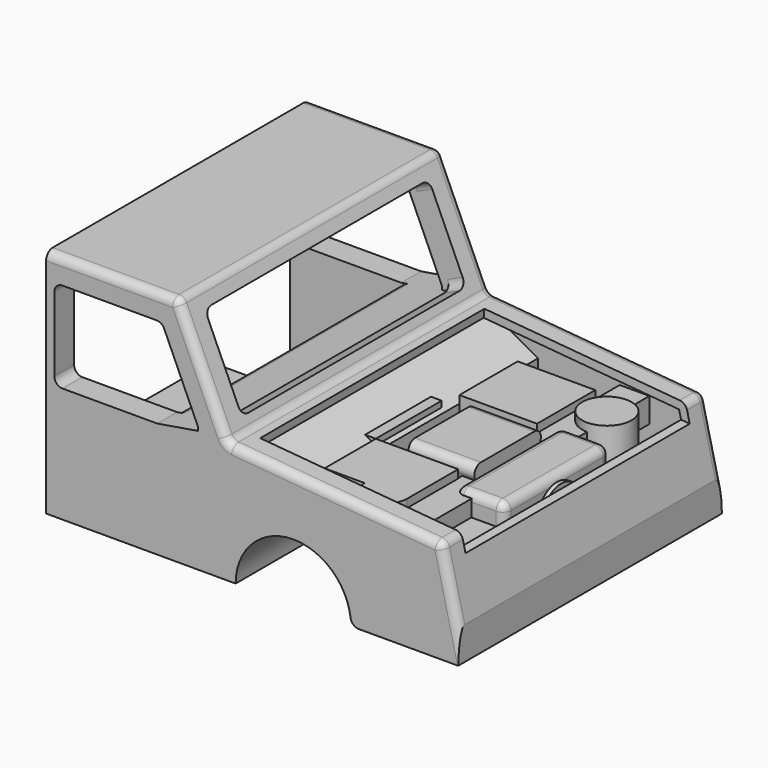
from build123d import *

# Parameters (mm, degrees)
F1_DEPTH       = 1000
F3_DEPTH       = 850
F4_W           = 1500
F4_H           = 1700
F5_DEPTH       = 100
F7_DEPTH       = 950
F9_DEPTH       = 400
F10_R          = 50
F11_R          = 150
F12_DEPTH      = 25
F13_R          = 50
F15_DEPTH      = 270
F17_DEPTH      = 1000
F18_W          = 600
F18_H          = 250
F19_DEPTH      = 250
F20_R          = 350
F21_DEPTH      = 1310
F22_R          = 50
F24_DEPTH      = 1380
F26_DEPTH      = 400
F28_DEPTH      = 150
F29_R          = 105
F30_DEPTH      = 1225
F30_DEPTH_BACK = 25
F31_W          = 180
F31_H          = 150
F32_DEPTH      = 1950
F33_R          = 150
F33_W          = 470.87931633
F33_H          = 441.7398571968
F34_DEPTH      = 180
F34_DEPTH_BACK = 50
F35_W          = 455.6799697876
F35_H          = 409.935683012
F36_DEPTH      = 100
F36_DEPTH_BACK = 50


with BuildPart() as f1:
    # F0 (on Front) → F1 (new body, symmetric)
    with BuildSketch(Plane.XZ):
        with BuildLine():
            Line((767.6470588235, 1700), (0, 1700))
            Line((0, 1700), (0, 300))
            Line((0, 300), (1103.1373033403, 300))
            ThreePointArc((1103.1373033403, 300), (1136.2091947286, 312.5), (1152.7451404228, 343.75))
            ThreePointArc((1152.7451404228, 343.75), (1500, 650), (1847.2548595772, 343.75))
            ThreePointArc((1847.2548595772, 343.75), (1863.7908052714, 312.5), (1896.8626966597, 300))
            Line((1896.8626966597, 300), (2500, 300))
            Line((2500, 300), (2500, 500))
            Line((2500, 500), (2408.3761577886, 883.3611142393))
            ThreePointArc((2408.3761577886, 883.3611142393), (2392.4030745749, 909.6000062773), (2364.1035813021, 921.5481242564))
            Line((2364.1035813021, 921.5481242564), (1129.229325017, 1029.5856225614))
            ThreePointArc((1129.229325017, 1029.5856225614), (1104.6193241933, 1038.6416182431), (1087.9773560568, 1058.9075525879))
            Line((1087.9773560568, 1058.9075525879), (813.2568149211, 1670.487804878))
            ThreePointArc((813.2568149211, 1670.487804878), (794.8096227314, 1691.9785078576), (767.6470588235, 1700))
        make_face()
        with BuildLine():
            ThreePointArc((50, 1500), (64.6446609407, 1535.3553390593), (100, 1550))
            Line((100, 1550), (670.5882352941, 1550))
            ThreePointArc((670.5882352941, 1550), (697.750799202, 1541.9785078576), (716.1979913917, 1520.487804878))
            Line((716.1979913917, 1520.487804878), (918.3370288248, 1070.487804878))
            ThreePointArc((918.3370288248, 1070.487804878), (914.7057805849, 1022.8374360921), (872.7272727273, 1000))
            Line((872.7272727273, 1000), (100, 1000))
            ThreePointArc((100, 1000), (64.6446609407, 1014.6446609407), (50, 1050))
            Line((50, 1050), (50, 1500))
        make_face(mode=Mode.SUBTRACT)
    extrude(amount=F1_DEPTH, both=True)

    # F2 (on Front) → F3 (cut, symmetric)
    with BuildSketch(Plane.XZ):
        Polygon((735.2941176471, 1600), (0, 1600), (0, 300), (2444.9838573448, 300), (2319.4915883295, 825.0691841445), (1032.8257756913, 937.6378564967), align=None)
    extrude(amount=F3_DEPTH, both=True, mode=Mode.SUBTRACT)

    # F4 (on face) → F5 (cut)
    with BuildSketch(Plane(origin=(97.9705989607, 0, 1119.8090702535), x_dir=(0.9961946981, 0, -0.0871557427), z_dir=(0.0871557427, 0, 0.9961946981))):
        with Locations((1835.197966855, 0)):
            Rectangle(F4_W, F4_H)
    extrude(amount=-F5_DEPTH, mode=Mode.SUBTRACT)

    # F6 (on Front) → F7 (cut, symmetric)
    with BuildSketch(Plane.XZ):
        Polygon((2359.7457941648, 871.7383893518), (1110.5418587764, 981.0295721303), (1110.5418587764, 281.0295721303), (2410.5418587764, 281.0295721303), (2410.5418587764, 450), (2460.5418587764, 450), align=None)
    extrude(amount=F7_DEPTH, both=True, mode=Mode.SUBTRACT)

    # F13
    f13_edges = [f1.edges().sort_by_distance(p)[0] for p in [
        (950.617085, -1000, 1364.697679),
        (1746.666453, 1000, 975.566873),
    ]]
    fillet(f13_edges, radius=F13_R)

    # F14 (on face) → F15 (cut)
    with BuildSketch(Plane(origin=(1301.1017251636, 0, 584.4521118382), x_dir=(0, 1, 0), z_dir=(0.912195122, 0, 0.4097560976))):
        with BuildLine():
            ThreePointArc((-850, 620.1249484155), (-835.3553390593, 584.7696093561), (-800, 570.1249484155))
            Line((-800, 570.1249484155), (800, 570.1249484155))
            ThreePointArc((800, 570.1249484155), (835.3553390593, 584.7696093561), (850, 620.1249484155))
            Line((850, 620.1249484155), (850, 1070.1249484155))
            ThreePointArc((850, 1070.1249484155), (835.3553390593, 1105.4802874748), (800, 1120.1249484155))
            Line((800, 1120.1249484155), (-800, 1120.1249484155))
            ThreePointArc((-800, 1120.1249484155), (-835.3553390593, 1105.4802874748), (-850, 1070.1249484155))
            Line((-850, 1070.1249484155), (-850, 620.1249484155))
        make_face()
    extrude(amount=-F15_DEPTH, mode=Mode.SUBTRACT)

    # F16 (on Front) → F17 (join, symmetric)
    with BuildSketch(Plane.XZ):
        Polygon((1424.8715378796, 800), (974.8715378796, 1050), (674.8715378796, 1000), (674.8715378796, 800), (1174.8715378796, 800), (1174.8715378796, 600), (1174.8715378796, 400), (1424.8715378796, 400), align=None)
        Polygon((1424.8715378796, 300), (1424.8715378796, 400), (1174.8715378796, 400), (1024.8715378796, 400), (0, 400), (0, 300), align=None)
        Polygon((1024.8715378796, 400), (1174.8715378796, 400), (1174.8715378796, 600), align=None)
    extrude(amount=F17_DEPTH, both=True)

    # F18 (on Front) → F19 (join, symmetric)
    with BuildSketch(Plane.XZ):
        Polygon((0, 300), (1400, 300), (1400, 600), (800, 600), (0, 600), align=None)
        with Locations((1100, 725)):
            Rectangle(F18_W, F18_H)
    extrude(amount=F19_DEPTH, both=True)

    # F20 (on Front) → F21 (cut, symmetric)
    with BuildSketch(Plane.XZ):
        with Locations((1500, 300)):
            Circle(F20_R)
    extrude(amount=F21_DEPTH, both=True, mode=Mode.SUBTRACT)

    # F22
    f22_edges = [f1.edges().sort_by_distance(p)[0] for p in [
        (674.871538, 0, 800),
        (674.871538, 0, 1000),
    ]]
    fillet(f22_edges, radius=F22_R)

    # F23 (on face) → F24 (cut)
    with BuildSketch(Plane(origin=(0, 0, 0), x_dir=(0, -1, 0), z_dir=(-1, 0, 0))):
        with BuildLine():
            Line((-150, 450), (-150, 300))
            Line((-150, 300), (150, 300))
            Line((150, 300), (150, 450))
            ThreePointArc((150, 450), (135.3553390593, 485.3553390593), (100, 500))
            Line((100, 500), (-100, 500))
            ThreePointArc((-100, 500), (-135.3553390593, 485.3553390593), (-150, 450))
        make_face()
    extrude(amount=-F24_DEPTH, mode=Mode.SUBTRACT)



with BuildPart() as f9:
    # F8 (on Front) → F9 (new body, symmetric)
    with BuildSketch(Plane.XZ):
        with BuildLine():
            Line((2250, 850), (2050, 850))
            ThreePointArc((2050, 850), (2014.6446609407, 835.3553390593), (2000, 800))
            Line((2000, 800), (2000, 500))
            ThreePointArc((2000, 500), (2014.6446609407, 464.6446609407), (2050, 450))
            Line((2050, 450), (2250, 450))
            ThreePointArc((2250, 450), (2285.3553390593, 464.6446609407), (2300, 500))
            Line((2300, 500), (2300, 800))
            ThreePointArc((2300, 800), (2285.3553390593, 835.3553390593), (2250, 850))
        make_face()
    extrude(amount=F9_DEPTH, both=True)

    # F10
    f10_edges = [f9.edges().sort_by_distance(p)[0] for p in [
        (2150, -400, 850),
        (2150, 400, 850),
    ]]
    fillet(f10_edges, radius=F10_R)

    # F11 (on face) → F12 (join, symmetric)
    with BuildSketch(Plane.YZ.offset(2300)):
        with Locations((0, 660)):
            Circle(F11_R)
    extrude(amount=F12_DEPTH, both=True)

    # F25 (on face) → F26 (join)
    with BuildSketch(Plane(origin=(2000, 0, 0), x_dir=(0, -1, 0), z_dir=(-1, 0, 0))):
        with BuildLine():
            Line((150, 900), (-150, 900))
            Line((-150, 900), (-150, 600))
            ThreePointArc((-150, 600), (-147.5161737638, 572.8158414129), (-140.1469536255, 546.5319591766))
            ThreePointArc((-140.1469536255, 546.5319591766), (0, 450), (140.1469536255, 546.5319591766))
            ThreePointArc((140.1469536255, 546.5319591766), (147.5161737638, 572.8158414129), (150, 600))
            Line((150, 600), (150, 900))
        make_face()
        with BuildLine():
            Line((-150, 600), (-150, 900))
            Line((-150, 900), (-202.4090390266, 900))
            ThreePointArc((-202.4090390266, 900), (-243.5863022536, 878.3625279751), (-249.1246902351, 832.1773197255))
            Line((-249.1246902351, 832.1773197255), (-140.1469536255, 546.5319591766))
            ThreePointArc((-140.1469536255, 546.5319591766), (-147.5161737638, 572.8158414129), (-150, 600))
        make_face()
        with BuildLine():
            Line((202.4090390266, 900), (150, 900))
            Line((150, 900), (150, 600))
            ThreePointArc((150, 600), (147.5161737638, 572.8158414129), (140.1469536255, 546.5319591766))
            Line((140.1469536255, 546.5319591766), (249.1246902351, 832.1773197255))
            ThreePointArc((249.1246902351, 832.1773197255), (243.5863022536, 878.3625279751), (202.4090390266, 900))
        make_face()
    extrude(amount=F26_DEPTH)

    # F27 (on Front) → F28 (join, symmetric)
    with BuildSketch(Plane.XZ):
        Polygon((1681.4885139465, 443.7106251717), (1660.2123975754, 704.3795585632), (1308.0242587981, 580.7129842787), (1216.2470817566, 473.7584888935), (1216.2470817566, 307.4244611528), align=None)
    extrude(amount=F28_DEPTH, both=True)


with BuildPart() as f1_1:
    add(f1.part)

    add(f9.part)  # F30 merges F9
    # F29 (on face) → F30 (join, two sides)
    with BuildSketch(Plane(origin=(1216.2470817566, 0, 0), x_dir=(0, -1, 0), z_dir=(-1, 0, 0))) as f30_sk:
        with Locations((0, 400)):
            Circle(F29_R)
    extrude(amount=F30_DEPTH)
    extrude(f30_sk.sketch, amount=-F30_DEPTH_BACK)

    # F31 (on face) → F32 (join)
    with BuildSketch(Plane.XZ.offset(-950)):
        with Locations((2010, 743.1786501513)):
            Rectangle(F31_W, F31_H)
    extrude(amount=F32_DEPTH)

    # F33 (on face) → F34 (join, two sides)
    with BuildSketch(Plane.XY.offset(818.1786501513)) as f34_sk:
        with Locations((2100, 627.4012327194)):
            Circle(F33_R)
        with Locations((1686.6853237152, 541.0294830799)):
            Rectangle(F33_W, F33_H)
        with BuildLine():
            Line((1422.2102165222, -665.217936039), (1665.0403738022, -665.217936039))
            ThreePointArc((1665.0403738022, -665.217936039), (1793.5826778412, -793.760240078), (1922.1249818802, -665.217936039))
            Line((1922.1249818802, -665.217936039), (1922.1249818802, -277.8724431992))
            Line((1922.1249818802, -277.8724431992), (1422.2102165222, -277.8724431992))
            Line((1422.2102165222, -277.8724431992), (1422.2102165222, -665.217936039))
        make_face()
    extrude(amount=-F34_DEPTH)
    extrude(f34_sk.sketch, amount=F34_DEPTH_BACK)

    # F35 (on face) → F36 (join, two sides)
    with BuildSketch(Plane(origin=(0, 0, 668.1786501513), x_dir=(1, 0, 0), z_dir=(0, 0, -1))) as f36_sk:
        with Locations((2147.8399848938, 586.2611681223)):
            Rectangle(F35_W, F35_H)
    extrude(amount=F36_DEPTH)
    extrude(f36_sk.sketch, amount=-F36_DEPTH_BACK)


solid = f1_1.part
